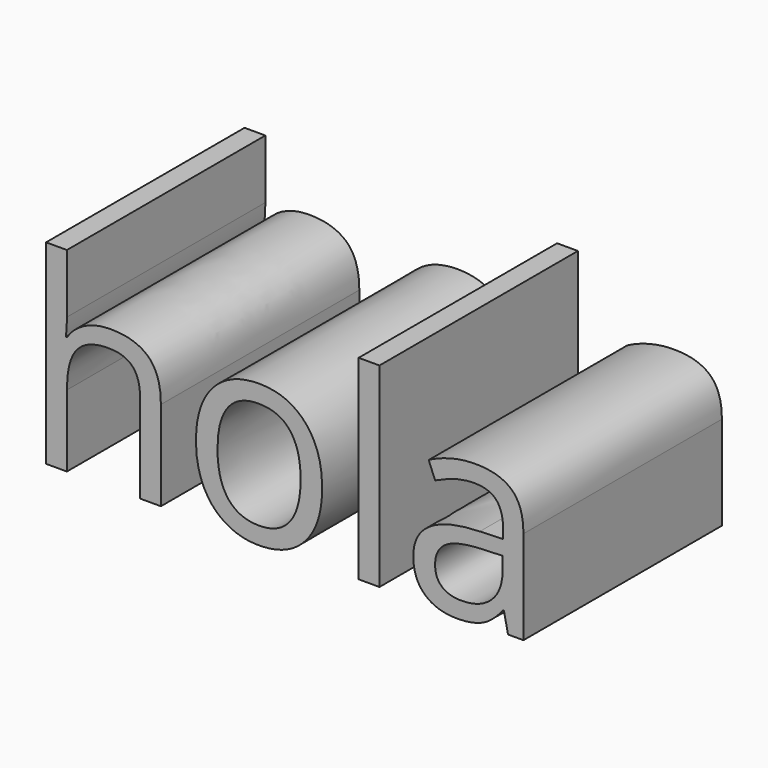
from build123d import *

# Parameters (mm, degrees)
F0_TEXT_SIZE = 26.2813694361
F1_DEPTH     = 25.4


# Not quite as in the source:
# - Text() gives the source's letters only with a copy of the font that has no kerning and outlines rounded to 1/6400 em; it was checked with that copy


with BuildPart() as f1:
    # F0 (on Front) → F1 (new body)
    with BuildSketch(Plane.XZ):
        with Locations((0, 0)):
            Text('hola', F0_TEXT_SIZE, font='Open Sans', text_align=(TextAlign.LEFT, TextAlign.BOTTOM))
    extrude(amount=F1_DEPTH)


solid = f1.part
